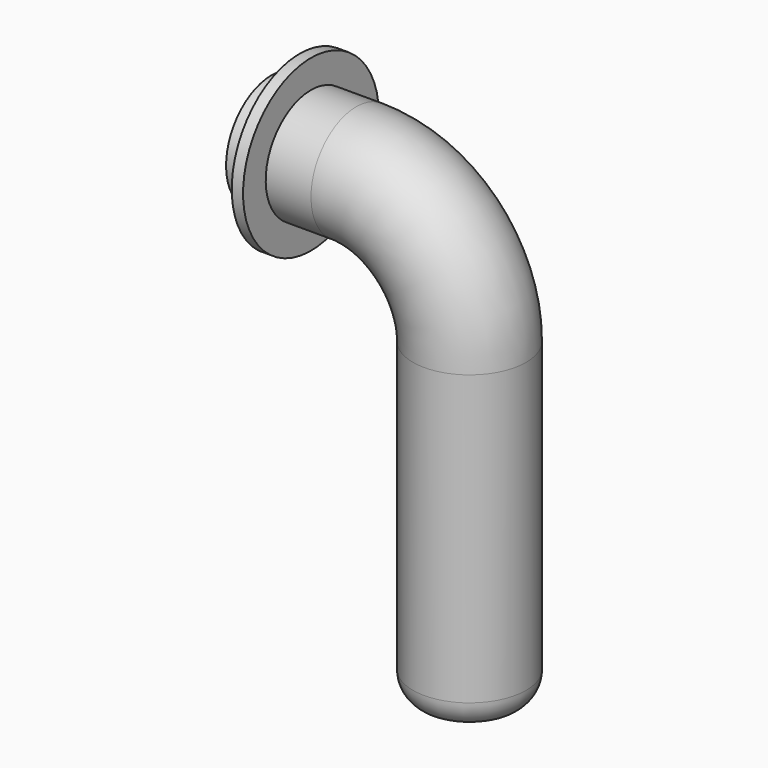
from build123d import *

# Parameters (mm, degrees)
F2_R     = 10
F2_R_2   = 8
F7_R     = 15
F7_R_2   = 10
F8_DEPTH = 2


# Not quite as in the source:
# - a fillet or chamfer that OpenCascade refuses, or shapes differently, is made with other operations: its cross-section is extruded or revolved along the edge and cut away or added


with BuildPart() as f3:
    # F3: sweep along a path in F0
    with BuildLine(Plane.XZ) as f3_path:
        Line((0, -45), (0, 10))
        ThreePointArc((0, 10), (-5.8578643763, 24.1421356237), (-20, 30))
        Line((-20, 30), (-35, 30))
    # F2 (on plane+point) → F3 (sweep)
    with BuildSketch(Plane.XY.offset(-45)):
        Circle(F2_R)
        Circle(F2_R_2, mode=Mode.SUBTRACT)
    sweep(path=f3_path.line)

    # F4: fillet of radius 5 on 1 edges, made by hand

    # F4_s1 → F4_t2 (revolve, cut)
    with BuildSketch(Plane.XZ):
        with BuildLine():
            ThreePointArc((10, -41), (9.472135955, -43.2360679775), (8, -45))
            Line((8, -45), (10, -45))
            Line((10, -45), (10, -41))
        make_face()
    revolve(axis=Axis((0, 0, -45), (0, 0, 1)), mode=Mode.SUBTRACT)

    # F5: fillet of radius 5 on 1 edges, made by hand

    # F5_s1 → F5_t2 (revolve, cut)
    with BuildSketch(Plane.XZ):
        with BuildLine():
            ThreePointArc((-35, 40), (-33.2360679775, 38.527864045), (-31, 38))
            Line((-31, 38), (-35, 38))
            Line((-35, 38), (-35, 40))
        make_face()
    revolve(axis=Axis((-35, 0, 30), (-1, 0, 0)), mode=Mode.SUBTRACT)

    # F7 (on offset) → F8 (join)
    with BuildSketch(Plane.YZ.offset(-30)):
        with Locations((0, 30)):
            Circle(F7_R)
        with Locations((0, 30)):
            Circle(F7_R_2, mode=Mode.SUBTRACT)
    extrude(amount=F8_DEPTH)


solid = f3.part
